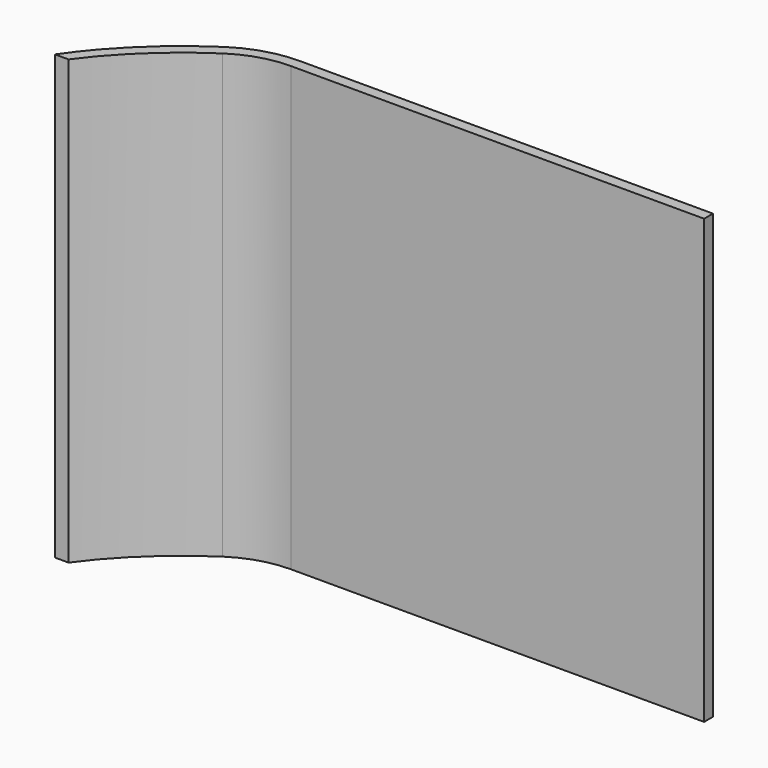
from build123d import *

# Parameters (mm, degrees)
F0_W     = 101.6
F0_H     = 101.6
F1_DEPTH = 12.7
F3_DEPTH = 101.6
F4_R     = 25.4
F5_T     = -2.54


# Not quite as in the source:
# - a feature of the source that left no trace in its solid (it failed there, or was rolled back) is left out


with BuildPart() as f1:
    # F0 (on Front) → F1 (new body, symmetric)
    with BuildSketch(Plane.XZ):
        with Locations((1.211412394, -8.554763478)):
            Rectangle(F0_W, F0_H)
    extrude(amount=F1_DEPTH, both=True)

    # F2 (on face) → F3 (join)
    with BuildSketch(Plane.XY.offset(42.245236522)):
        with BuildLine():
            Line((-49.588587606, -12.7), (-49.588587606, 12.7))
            add(Edge.make_bspline(
                [(-49.588587606, 12.7), (-67.7978310293, 3.2621913661), (-78.5642321364, -12.7)],
                knots=[1.1900846756, 1.1900846756, 1.1900846756, 2.1282604502, 2.1282604502, 2.1282604502], degree=2, weights=[1, 0.8919810006, 1]))
            Line((-78.5642321364, -12.7), (-49.588587606, -12.7))
        make_face()
    extrude(amount=-F3_DEPTH)

    # F4
    f4_edges = [f1.edges().sort_by_distance(p)[0] for p in [
        (-49.588588, 12.7, -8.554763),
    ]]
    fillet(f4_edges, radius=F4_R)

    # F5
    f5_openings = [f1.faces().sort_by_distance(p)[0] for p in [
        (-7.437576, -0.524073, 42.245237),
        (-13.27641, -12.7, -8.554763),
        (52.011412, 0, -8.554763),
        (-7.437576, -0.524073, -59.354763),
    ]]
    offset(amount=F5_T, openings=f5_openings)


solid = f1.part
